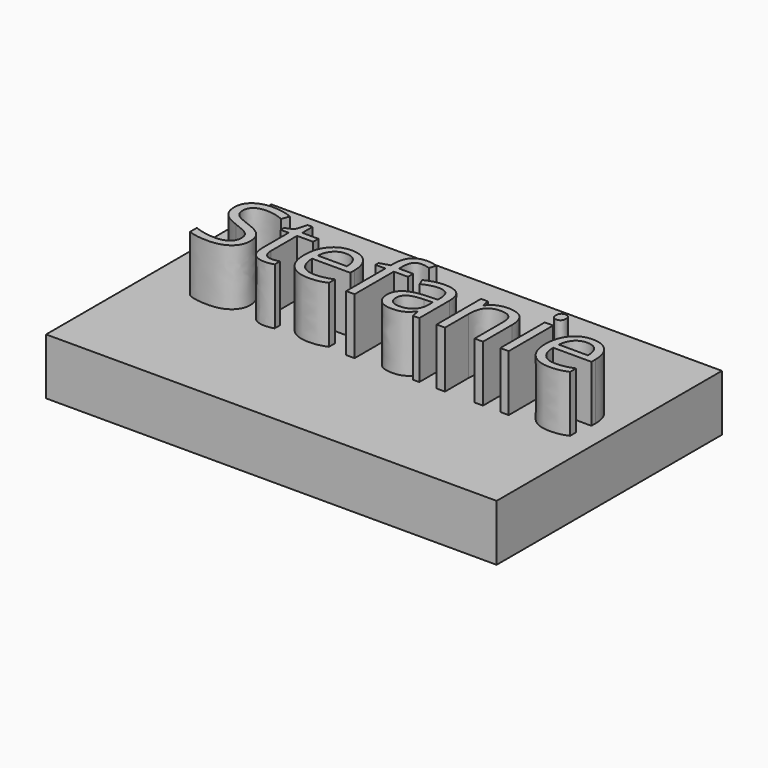
from build123d import *

# Parameters (mm, degrees)
F0_W         = 101.6
F0_H         = 63.5
F1_DEPTH     = 6.35
F2_TEXT_SIZE = 23.4053231314
F3_DEPTH     = 12.7


# Not quite as in the source:
# - Text() gives the source's letters only with a copy of the font that has no kerning and outlines rounded to 1/6400 em; it was checked with that copy


with BuildPart() as f1:
    # F0 (on Top) → F1 (new body, symmetric)
    with BuildSketch(Plane.XY):
        Rectangle(F0_W, F0_H)
    extrude(amount=F1_DEPTH, both=True)

    # F2 (on face) → F3 (join)
    with BuildSketch(Plane.XY.offset(6.35)):
        with Locations((-41.4290465415, -4.8944517339)):
            Text('Stefanie', F2_TEXT_SIZE, font='Open Sans', text_align=(TextAlign.LEFT, TextAlign.BOTTOM))
    extrude(amount=F3_DEPTH)


solid = f1.part
